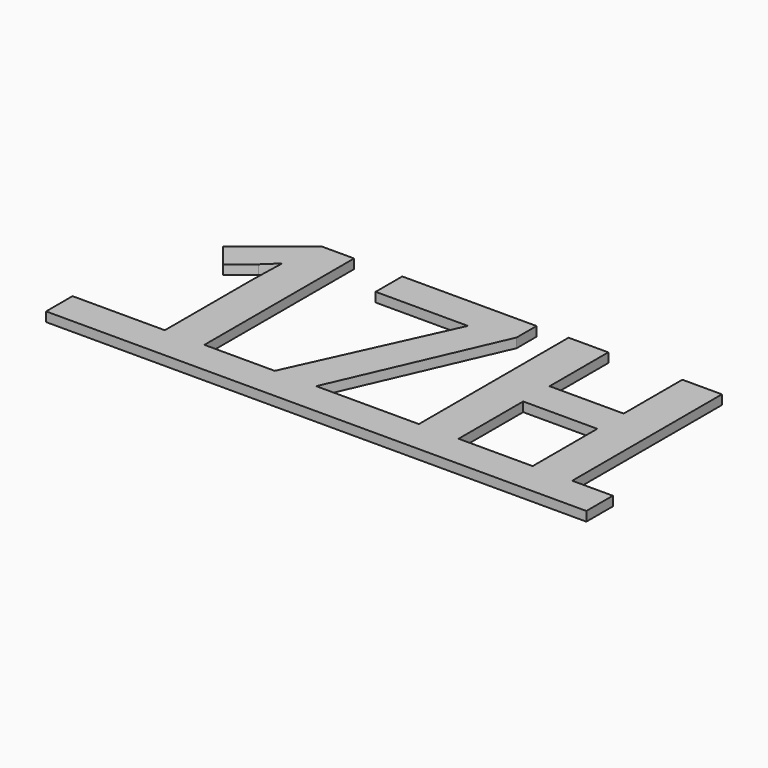
from build123d import *

# Parameters (mm, degrees)
F0_TEXT_SIZE = 1411.1111111111
F1_DEPTH     = 50.8


# Not quite as in the source:
# - a feature names something its author has since deleted; it is built from what else it names
# - Text() gives the source's letters only with a copy of the font that has no kerning and outlines rounded to 1/6400 em; it was checked with that copy


with BuildPart() as f1:
    # F0 (on Top) → F1 (new body)
    with BuildSketch(Plane.XY):
        Polygon((-275.5148668289, 0), (-275.5148668289, -177.8), (2633.1379109489, -177.8), (2633.1379109489, 0), (2414.6361748377, 0), (2201.6465915044, 0), (1802.7872165044, 0), (1589.1361748377, 0), (1036.5979803933, 0), (813.2455498377, 0), (434.4504109489, 0), (221.4608276155, 0), align=None)
        with Locations((-148.5148668289, 0)):
            Text('17H', F0_TEXT_SIZE, font='Open Sans', font_style=FontStyle.BOLD, text_align=(TextAlign.LEFT, TextAlign.BOTTOM))
    extrude(amount=F1_DEPTH)


solid = f1.part
